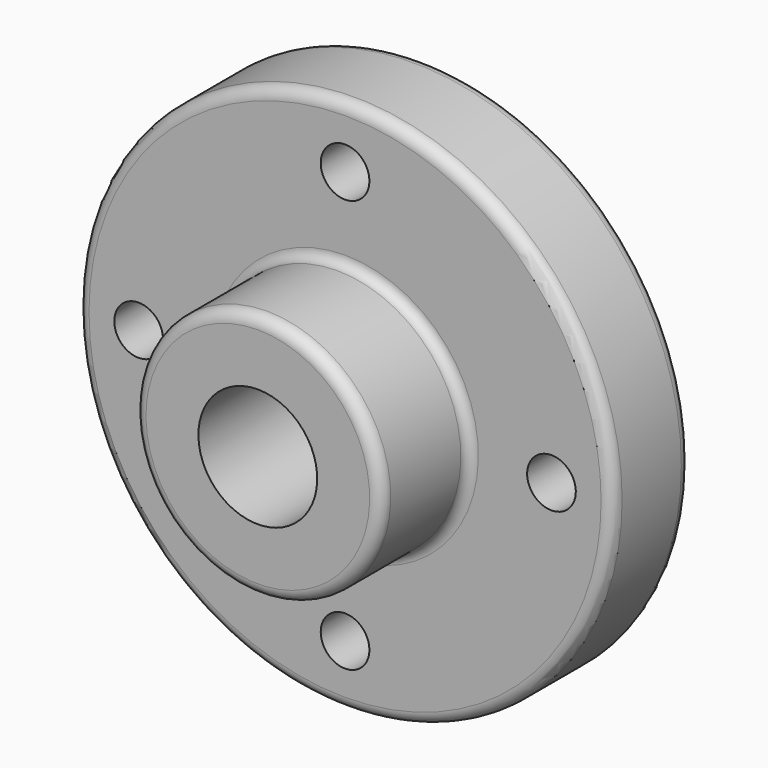
from build123d import *

# Parameters (mm, degrees)
F0_R            = 69.85
F1_DEPTH        = 25.4
F2_R            = 19.05
F2_R_2          = 6.35
F3_DEPTH        = 25.401
F3_COPIES_COUNT = 4
F6_R            = 3.048
F7_R            = 3.048
F8_R            = 2.54


# Not quite as in the source:
# - a pattern or mirror of a feature is missing from the dataset's text; its kind, count and spacing are read off the source's solid


with BuildPart() as f1:
    # F0 (on Front) → F1 (new body)
    with BuildSketch(Plane.XZ):
        Circle(F0_R)
    extrude(amount=F1_DEPTH)

    # F2 (on Front) → F3 (cut, through all)
    with BuildSketch(Plane.XZ):
        Circle(F2_R)
        with Locations((0, 53.848)):
            Circle(F2_R_2)
    f3 = extrude(amount=F3_DEPTH, mode=Mode.SUBTRACT)

    # F3_copies: F3 ×4 about axis
    f3_copies_axis = Axis((0, 0, 0), (0, 1, 0))
    for i in range(1, F3_COPIES_COUNT):
        add(f3.rotate(f3_copies_axis, i * 360 / F3_COPIES_COUNT), mode=Mode.SUBTRACT)

    # F4 (on Right) → F5 (revolve)
    with BuildSketch(Plane.YZ):
        with BuildLine():
            Line((-53.848, 15.4953468409), (0, 15.4953468409))
            Line((0, 15.4953468409), (0, 32.2310491102))
            Line((0, 32.2310491102), (-25.3001134843, 32.2310491102))
            Line((-25.3001134843, 32.2310491102), (-50.8, 32.2310491102))
            ThreePointArc((-50.8, 32.2310491102), (-52.9552614691, 31.3383105793), (-53.848, 29.1830491102))
            Line((-53.848, 29.1830491102), (-53.848, 15.4953468409))
        make_face()
    revolve(axis=Axis((0, -22.6452342175, 0), (0, -1, 0)))

    # F6
    f6_edges = [f1.edges().sort_by_distance(p)[0] for p in [
        (-69.85, -25.4, 0),
    ]]
    fillet(f6_edges, radius=F6_R)

    # F7
    f7_edges = [f1.edges().sort_by_distance(p)[0] for p in [
        (-69.85, 0, 0),
    ]]
    fillet(f7_edges, radius=F7_R)

    # F8
    f8_edges = [f1.edges().sort_by_distance(p)[0] for p in [
        (0, -25.4, -32.231049),
    ]]
    fillet(f8_edges, radius=F8_R)


solid = f1.part
